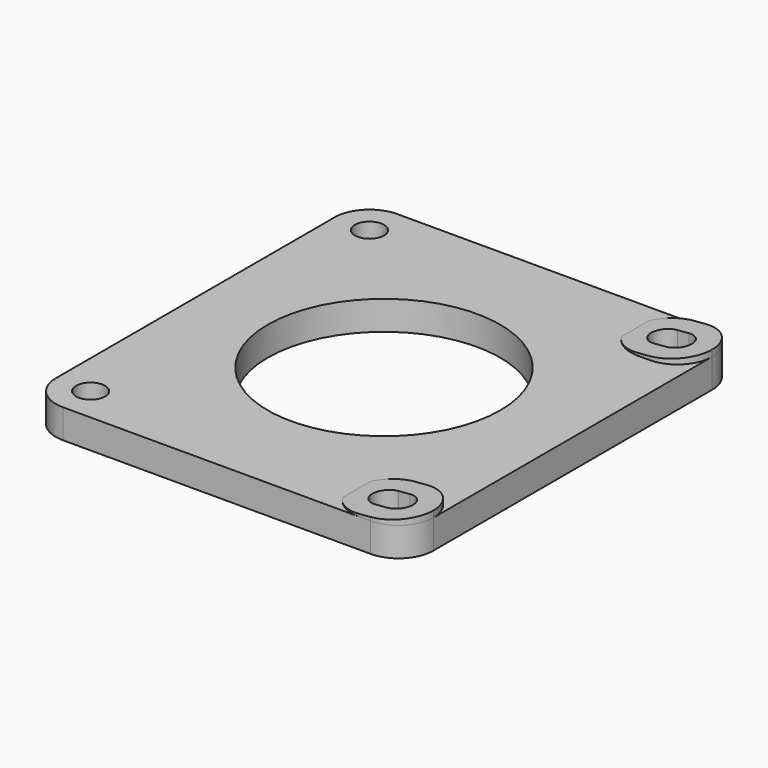
from build123d import *

# Parameters (mm, degrees)
F0_W        = 65
F0_H        = 72
F0_R        = 2.5
F0_R_2      = 20
F1_DEPTH    = 5
F3_DEPTH    = 1.1
F5_DEPTH    = 72.001
F6_T1_DEPTH = 35


# Not quite as in the source:
# - a fillet or chamfer that OpenCascade refuses, or shapes differently, is made with other operations: its cross-section is extruded or revolved along the edge and cut away or added


with BuildPart() as f1:
    # F0 (on Top) → F1 (new body)
    with BuildSketch(Plane.XY):
        Rectangle(F0_W, F0_H)
        with Locations((-26.5, -30)):
            Circle(F0_R, mode=Mode.SUBTRACT)
        with BuildLine():
            Line((26.5, -32.5), (24.5, -32.5))
            ThreePointArc((24.5, -32.5), (22, -30), (24.5, -27.5))
            Line((24.5, -27.5), (26.5, -27.5))
            ThreePointArc((26.5, -27.5), (29, -30), (26.5, -32.5))
        make_face(mode=Mode.SUBTRACT)
        with Locations((-26.5, 30)):
            Circle(F0_R, mode=Mode.SUBTRACT)
        Circle(F0_R_2, mode=Mode.SUBTRACT)
        with BuildLine():
            Line((26.5, 27.5), (24.5, 27.5))
            ThreePointArc((24.5, 27.5), (22, 30), (24.5, 32.5))
            Line((24.5, 32.5), (26.5, 32.5))
            ThreePointArc((26.5, 32.5), (29, 30), (26.5, 27.5))
        make_face(mode=Mode.SUBTRACT)
    extrude(amount=F1_DEPTH)

    # F2 (on face) → F3 (join)
    with BuildSketch(Plane.XY.offset(5)):
        with BuildLine():
            Line((26.5, -24.0000002086), (24.5, -24.0000002086))
            ThreePointArc((24.5, -24.0000002086), (18.5000002086, -30), (24.5, -35.9999997914))
            Line((24.5, -35.9999997914), (26.5, -35.9999997914))
            ThreePointArc((26.5, -35.9999997914), (30.7426405396, -34.2426405396), (32.4999997914, -30))
            ThreePointArc((32.4999997914, -30), (30.7426405396, -25.7573594604), (26.5, -24.0000002086))
        make_face()
        with BuildLine():
            ThreePointArc((26.5, -27.5), (29, -30), (26.5, -32.5))
            Line((26.5, -32.5), (24.5, -32.5))
            ThreePointArc((24.5, -32.5), (22, -30), (24.5, -27.5))
            Line((24.5, -27.5), (26.5, -27.5))
        make_face(mode=Mode.SUBTRACT)
        with BuildLine():
            ThreePointArc((26.5, 24.0000002086), (30.7426405396, 25.7573594604), (32.4999997914, 30))
            ThreePointArc((32.4999997914, 30), (30.7426405396, 34.2426405396), (26.5, 35.9999997914))
            Line((26.5, 35.9999997914), (24.5, 35.9999997914))
            ThreePointArc((24.5, 35.9999997914), (18.5000002086, 30), (24.5, 24.0000002086))
            Line((24.5, 24.0000002086), (26.5, 24.0000002086))
        make_face()
        with BuildLine():
            ThreePointArc((26.5, 32.5), (29, 30), (26.5, 27.5))
            Line((26.5, 27.5), (24.5, 27.5))
            ThreePointArc((24.5, 27.5), (22, 30), (24.5, 32.5))
            Line((24.5, 32.5), (26.5, 32.5))
        make_face(mode=Mode.SUBTRACT)
    extrude(amount=F3_DEPTH)

    # F4 (on face) → F5 (cut, through all)
    with BuildSketch(Plane.XZ.offset(36)):
        Polygon((19.295739324, 5), (32.5, 6.1), (18.5000002086, 6.1), (18.5000002086, 5), align=None)
    extrude(amount=-F5_DEPTH, mode=Mode.SUBTRACT)

    # F6: fillet of radius 6 on 4 edges, made by hand

    # F6_s2 → F6_t1 (cut)
    with BuildSketch(Plane.XY.offset(-15)):
        with BuildLine():
            ThreePointArc((-32.5, -30), (-30.7426406871, -34.2426406871), (-26.5, -36))
            Line((-26.5, -36), (-32.5, -36))
            Line((-32.5, -36), (-32.5, -30))
        make_face()
        with BuildLine():
            ThreePointArc((-32.5, 30), (-30.7426406871, 34.2426406871), (-26.5, 36))
            Line((-26.5, 36), (-32.5, 36))
            Line((-32.5, 36), (-32.5, 30))
        make_face()
        with BuildLine():
            ThreePointArc((32.5, 30), (30.7426406871, 34.2426406871), (26.5, 36))
            Line((26.5, 36), (32.5, 36))
            Line((32.5, 36), (32.5, 30))
        make_face()
        with BuildLine():
            ThreePointArc((32.5, -30), (30.7426406871, -34.2426406871), (26.5, -36))
            Line((26.5, -36), (32.5, -36))
            Line((32.5, -36), (32.5, -30))
        make_face()
    extrude(amount=F6_T1_DEPTH, mode=Mode.SUBTRACT)


solid = f1.part
